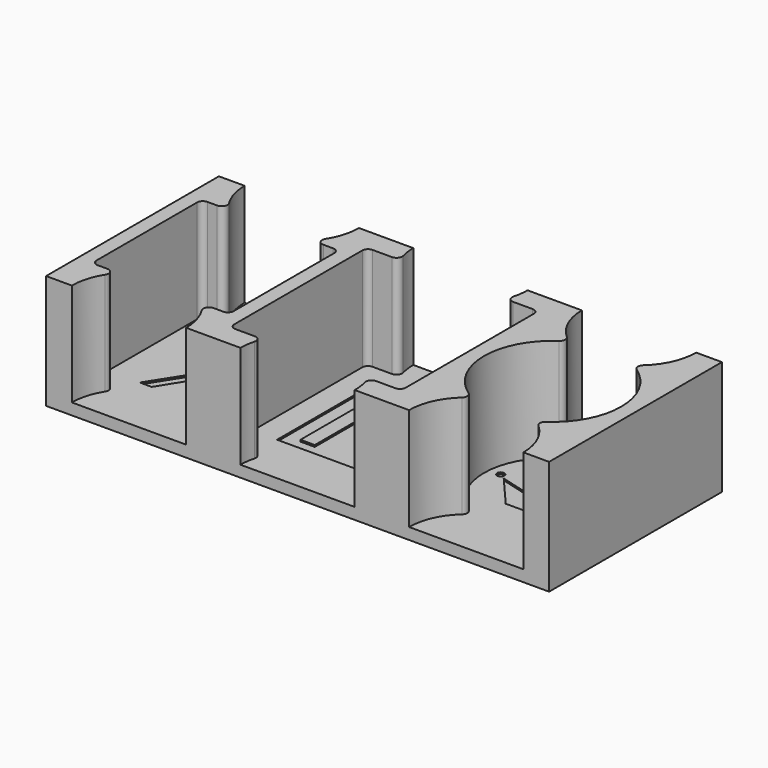
from build123d import *

# Parameters (mm, degrees)
F0_W         = 111.76
F0_H         = 48
F1_DEPTH     = 25.4
F3_DEPTH     = 22.86
F4_TEXT_SIZE = 29.9861111111
F4_W         = 27.2026264572
F4_H         = 25.4
F4_W_2       = 3.175
F4_H_2       = 20.32
F4_R         = 0.8001
F5_DEPTH     = 0.381
F6_R         = 1.27


# Not quite as in the source:
# - a feature names something its author has since deleted; it is built from what else it names
# - Text() gives the source's letters only with a copy of the font that has no kerning and outlines rounded to 1/6400 em; it was checked with that copy


with BuildPart() as f1:
    # F0 (on Top) → F1 (new body)
    with BuildSketch(Plane.XY):
        with Locations((55.88, 24)):
            Rectangle(F0_W, F0_H)
    extrude(amount=F1_DEPTH)

    # F2 (on face) → F3 (cut)
    with BuildSketch(Plane.XY.offset(25.4)):
        with BuildLine():
            Line((9.219762102, 39.24), (3.175, 39.24))
            Line((3.175, 39.24), (3.175, 8.76))
            Line((3.175, 8.76), (9.219762102, 8.76))
            ThreePointArc((9.219762102, 8.76), (18.415, 12.7), (27.610237898, 8.76))
            Line((27.610237898, 8.76), (33.655, 8.76))
            Line((33.655, 8.76), (33.655, 39.24))
            Line((33.655, 39.24), (27.610237898, 39.24))
            ThreePointArc((27.610237898, 39.24), (18.415, 35.3), (9.219762102, 39.24))
        make_face()
        with BuildLine():
            ThreePointArc((5.715, 48), (6.6236997896, 43.2824540969), (9.219762102, 39.24))
            Line((9.219762102, 39.24), (27.610237898, 39.24))
            ThreePointArc((27.610237898, 39.24), (30.2063002104, 43.2824540969), (31.115, 48))
            Line((31.115, 48), (5.715, 48))
        make_face()
        with BuildLine():
            Line((27.610237898, 39.24), (9.219762102, 39.24))
            ThreePointArc((9.219762102, 39.24), (18.415, 35.3), (27.610237898, 39.24))
        make_face()
        with BuildLine():
            ThreePointArc((27.610237898, 8.76), (18.415, 12.7), (9.219762102, 8.76))
            Line((9.219762102, 8.76), (27.610237898, 8.76))
        make_face()
        with BuildLine():
            Line((27.610237898, 8.76), (9.219762102, 8.76))
            ThreePointArc((9.219762102, 8.76), (6.6236997896, 4.7175459031), (5.715, 0))
            Line((5.715, 0), (31.115, 0))
            ThreePointArc((31.115, 0), (30.2063002104, 4.7175459031), (27.610237898, 8.76))
        make_face()
        with BuildLine():
            Line((68.58, 48), (43.18, 48))
            ThreePointArc((43.18, 48), (43.4336278531, 45.4745653088), (44.1843811622, 43.05))
            Line((44.1843811622, 43.05), (67.5756188378, 43.05))
            ThreePointArc((67.5756188378, 43.05), (68.3263721469, 45.4745653088), (68.58, 48))
        make_face()
        with BuildLine():
            ThreePointArc((67.5756188378, 43.05), (55.88, 35.3), (44.1843811622, 43.05))
            Line((44.1843811622, 43.05), (36.83, 43.05))
            Line((36.83, 43.05), (36.83, 4.95))
            Line((36.83, 4.95), (44.1843811622, 4.95))
            ThreePointArc((44.1843811622, 4.95), (55.88, 12.7), (67.5756188378, 4.95))
            Line((67.5756188378, 4.95), (74.93, 4.95))
            Line((74.93, 4.95), (74.93, 43.05))
            Line((74.93, 43.05), (67.5756188378, 43.05))
        make_face()
        with BuildLine():
            Line((67.5756188378, 43.05), (44.1843811622, 43.05))
            ThreePointArc((44.1843811622, 43.05), (55.88, 35.3), (67.5756188378, 43.05))
        make_face()
        with BuildLine():
            ThreePointArc((44.1843811622, 4.95), (43.4336278531, 2.5254346912), (43.18, 0))
            Line((43.18, 0), (68.58, 0))
            ThreePointArc((68.58, 0), (68.3263721469, 2.5254346912), (67.5756188378, 4.95))
            Line((67.5756188378, 4.95), (44.1843811622, 4.95))
        make_face()
        with BuildLine():
            Line((106.045, 48), (80.645, 48))
            ThreePointArc((80.645, 48), (82.128518064, 42.0434462162), (86.2324855085, 37.4784916667))
            ThreePointArc((86.2324855085, 37.4784916667), (93.345, 39.24), (100.4575144915, 37.4784916667))
            ThreePointArc((100.4575144915, 37.4784916667), (104.561481936, 42.0434462162), (106.045, 48))
        make_face()
        with BuildLine():
            ThreePointArc((67.5756188378, 4.95), (55.88, 12.7), (44.1843811622, 4.95))
            Line((44.1843811622, 4.95), (67.5756188378, 4.95))
        make_face()
        with BuildLine():
            ThreePointArc((100.4575144915, 37.4784916667), (93.345, 35.3), (86.2324855085, 37.4784916667))
            ThreePointArc((86.2324855085, 37.4784916667), (78.105, 24), (86.2324855085, 10.5215083333))
            ThreePointArc((86.2324855085, 10.5215083333), (93.345, 12.7), (100.4575144915, 10.5215083333))
            ThreePointArc((100.4575144915, 10.5215083333), (106.3959064982, 16.1303469216), (108.585, 24))
            ThreePointArc((108.585, 24), (106.3959064982, 31.8696530784), (100.4575144915, 37.4784916667))
        make_face()
        with BuildLine():
            ThreePointArc((100.4575144915, 37.4784916667), (93.345, 39.24), (86.2324855085, 37.4784916667))
            ThreePointArc((86.2324855085, 37.4784916667), (93.345, 35.3), (100.4575144915, 37.4784916667))
        make_face()
        with BuildLine():
            ThreePointArc((86.2324855085, 10.5215083333), (82.128518064, 5.9565537838), (80.645, 0))
            Line((80.645, 0), (106.045, 0))
            ThreePointArc((106.045, 0), (104.561481936, 5.9565537838), (100.4575144915, 10.5215083333))
            ThreePointArc((100.4575144915, 10.5215083333), (93.345, 8.76), (86.2324855085, 10.5215083333))
        make_face()
        with BuildLine():
            ThreePointArc((100.4575144915, 10.5215083333), (93.345, 12.7), (86.2324855085, 10.5215083333))
            ThreePointArc((86.2324855085, 10.5215083333), (93.345, 8.76), (100.4575144915, 10.5215083333))
        make_face()
    extrude(amount=-F3_DEPTH, mode=Mode.SUBTRACT)

    # F4 (on face) → F5 (cut)
    with BuildSketch(Plane.XY.offset(2.54)):
        with Locations((10.1464904159, 13.205)):
            Text('X', F4_TEXT_SIZE, font='Open Sans', text_align=(TextAlign.LEFT, TextAlign.BOTTOM))
        with Locations((55.88, 24)):
            Rectangle(F4_W, F4_H)
        with Locations((47.0411867714, 24)):
            Rectangle(F4_W_2, F4_H_2, mode=Mode.SUBTRACT)
        Polygon((82.062110968, 24.5173185093), (88.2906497618, 17.2985749907), (98.3993502382, 17.2985749907), (104.627889032, 24.5173185093), (98.7550836471, 22.9156460174), (100.0335352135, 27.603306748), (93.345, 24.0189385936), (86.6564647865, 27.603306748), (87.9349163529, 22.9156460174), align=None)
        with Locations((85.785248209, 28.945551776)):
            Circle(F4_R)
        with Locations((80.7141832355, 25.3797168325)):
            Circle(F4_R)
        Polygon((93.345, 31.2579385936), (91.7575, 27.0645730197), (93.345, 24.9079385936), (94.9325, 27.0645730197), align=None)
        with Locations((93.345, 32.8581385936)):
            Circle(F4_R)
        with Locations((100.904751791, 28.945551776)):
            Circle(F4_R)
        with Locations((105.9758167645, 25.3797168325)):
            Circle(F4_R)
    extrude(amount=-F5_DEPTH, mode=Mode.SUBTRACT)

    # F6
    f6_edges = [f1.edges().sort_by_distance(p)[0] for p in [
        (33.655, 39.24, 13.97),
        (3.175, 39.24, 13.97),
        (33.655, 8.76, 13.97),
        (3.175, 8.76, 13.97),
        (36.83, 4.95, 13.97),
        (36.83, 43.05, 13.97),
        (74.93, 43.05, 13.97),
        (74.93, 4.95, 13.97),
        (86.232486, 10.521508, 13.97),
        (100.457514, 10.521508, 13.97),
        (86.232486, 37.478492, 13.97),
        (100.457514, 37.478492, 13.97),
        (67.575619, 4.95, 13.97),
        (44.184381, 4.95, 13.97),
        (44.184381, 43.05, 13.97),
        (67.575619, 43.05, 13.97),
        (9.219762, 39.24, 13.97),
        (27.610238, 39.24, 13.97),
        (9.219762, 8.76, 13.97),
        (27.610238, 8.76, 13.97),
    ]]
    fillet(f6_edges, radius=F6_R)


solid = f1.part
